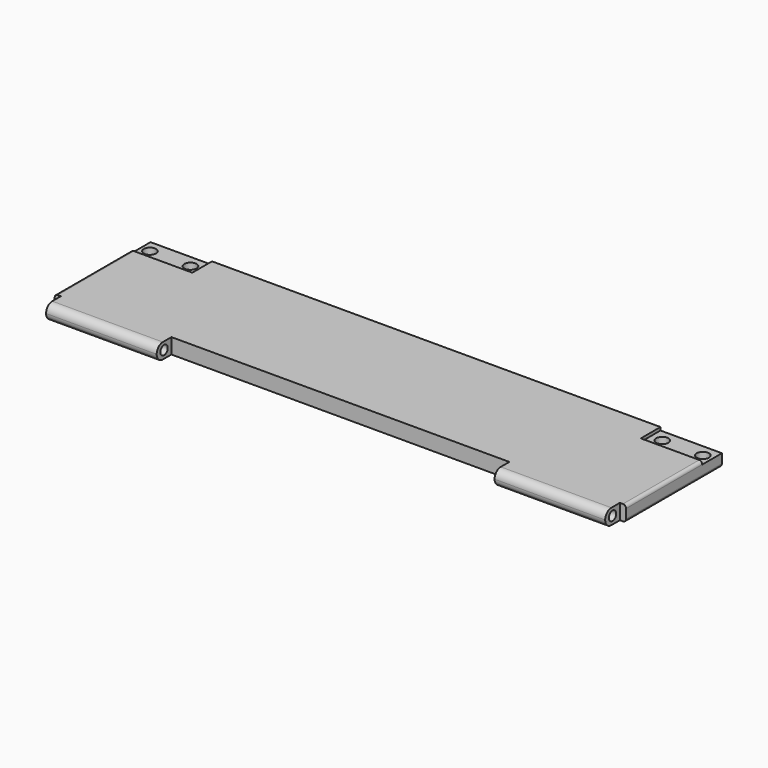
from build123d import *

# Parameters (mm, degrees)
F1_DEPTH  = 6.35
F2_W      = 25.4
F2_H      = 10.16
F3_DEPTH  = 1.27
F4_R      = 2.54
F5_DEPTH  = 25.4
F6_R      = 2.54
F7_DEPTH  = 25.4
F8_R      = 1.905
F9_DEPTH  = 254
F10_R     = 3.17499
F11_R     = 1.26999
F12_W     = 10.7186027977
F12_H     = 11.3617175813
F13_DEPTH = 2.54
F14_W     = 7.8115976844
F14_H     = 7.0746540246
F15_DEPTH = 2.54


# Not quite as in the source:
# - a fillet or chamfer is up to 0.001 mm smaller than in the source, because OpenCascade refuses the exact size


with BuildPart() as f1:
    # F0 (on Top) → F1 (new body)
    with BuildSketch(Plane.XY):
        Polygon((-53.3815915518, -2.0840423941), (-101.6415915518, -2.0840423941), (-101.6415915518, -51.6140423941), (-101.6415915518, -59.2340423941), (-53.3815915518, -59.2340423941), (-53.3815915518, -51.6140423941), (86.3184084482, -51.6140423941), (86.3184084482, -59.2340423941), (134.5784084482, -59.2340423941), (134.5784084482, -51.6140423941), (134.5784084482, -2.0840423941), (86.3184084482, -2.0840423941), align=None)
    extrude(amount=F1_DEPTH)

    # F2 (on face) → F3 (cut)
    with BuildSketch(Plane.XY.offset(6.35)):
        with Locations((-88.9415915518, -7.1640423941)):
            Rectangle(F2_W, F2_H)
        with Locations((121.8784084482, -7.1640423941)):
            Rectangle(F2_W, F2_H)
    extrude(amount=-F3_DEPTH, mode=Mode.SUBTRACT)

    # F4 (on face) → F5 (cut)
    with BuildSketch(Plane.XY.offset(5.08)):
        with Locations((-97.8315915518, -7.1640423941)):
            Circle(F4_R)
        with Locations((-81.0675915518, -7.1640423941)):
            Circle(F4_R)
    extrude(amount=-F5_DEPTH, mode=Mode.SUBTRACT)

    # F6 (on face) → F7 (cut)
    with BuildSketch(Plane.XY.offset(5.08)):
        with Locations((130.7684084482, -7.1640423941)):
            Circle(F6_R)
        with Locations((114.0044084482, -7.1640423941)):
            Circle(F6_R)
    extrude(amount=-F7_DEPTH, mode=Mode.SUBTRACT)

    # F8 (on face) → F9 (cut, symmetric)
    with BuildSketch(Plane.YZ.offset(-53.3815915518)):
        with Locations((-55.4240423941, 3.175)):
            Circle(F8_R)
    extrude(amount=F9_DEPTH, both=True, mode=Mode.SUBTRACT)

    # F10 (radius 3.175 in the source; OpenCascade refuses exactly that, so slightly less here)
    f10_edges = [f1.edges().sort_by_distance(p)[0] for p in [
        (-77.511592, -59.234042, 6.35),
        (-77.511592, -59.234042, 0),
        (110.448408, -59.234042, 6.35),
        (110.448408, -59.234042, 0),
    ]]
    fillet(f10_edges, radius=F10_R)

    # F11 (radius 1.27 in the source; OpenCascade refuses exactly that, so slightly less here)
    f11_edges = [f1.edges().sort_by_distance(p)[0] for p in [
        (-101.641592, -34.151547, 6.35),
        (134.578408, -34.151547, 6.35),
    ]]
    fillet(f11_edges, radius=F11_R)

    # F12 (on face) → F13 (cut)
    with BuildSketch(Plane(origin=(-101.6415915518, 0, 0), x_dir=(0, -1, 0), z_dir=(-1, 0, 0))):
        with Locations((56.973343793, 2.878480358)):
            Rectangle(F12_W, F12_H)
    extrude(amount=-F13_DEPTH, mode=Mode.SUBTRACT)

    # F14 (on face) → F15 (cut)
    with BuildSketch(Plane.YZ.offset(134.5784084482)):
        with Locations((-55.5198412363, 2.9937927611)):
            Rectangle(F14_W, F14_H)
    extrude(amount=-F15_DEPTH, mode=Mode.SUBTRACT)


solid = f1.part
